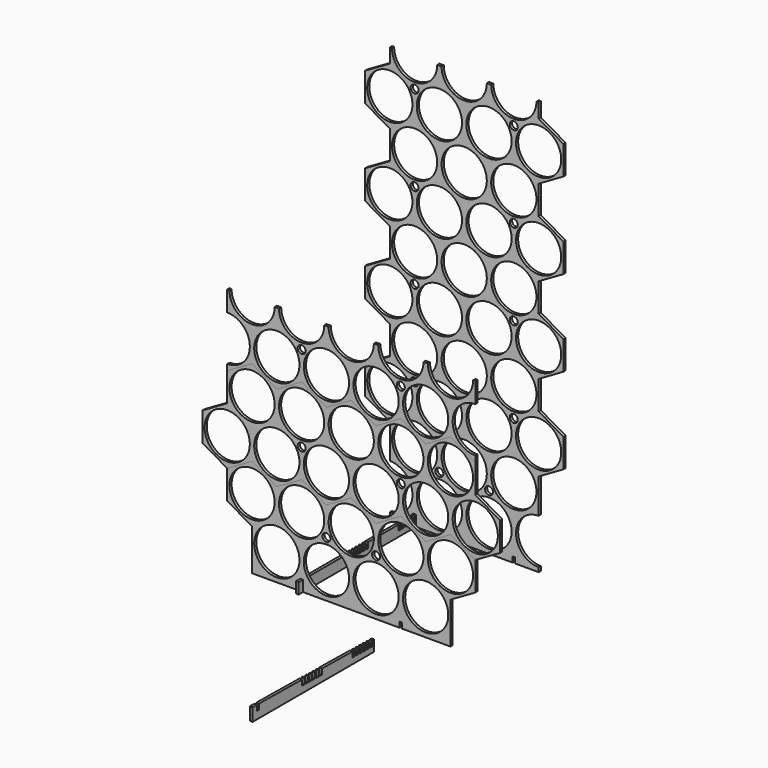
from build123d import *
from build123d import SkipClean  # not in build123d's __all__

# Parameters (mm, degrees)
F0_R           = 41.5
F1_DEPTH       = 5
F2_R           = 41.5
F3_DEPTH       = 5
F4_R           = 41.5
F5_DEPTH       = 5
F10_DEPTH      = 5
F11_R          = 41.5
F12_DEPTH      = 5
F13_R          = 7.25
F14_DEPTH      = 10.001
F14_DEPTH_BACK = 269.001
F16_DEPTH      = 5


with BuildPart() as f1:
    # F0 (on Front) → F1 (new body)
    with BuildSketch(Plane.XZ):
        with BuildLine():
            Line((-88.5, 0), (0, 0))
            Line((0, 0), (0, 86.8083117444))
            ThreePointArc((0, 86.8083117444), (-41.5, 128.3083117444), (0, 169.8083117444))
            Line((0, 169.8083117444), (0, 180.8471862406))
            Line((0, 180.8471862406), (-45.5, 154.5777489925))
            Line((-45.5, 154.5777489925), (-91, 180.8471862406))
            Line((-91, 180.8471862406), (-136.5, 154.5777489925))
            Line((-136.5, 154.5777489925), (-182, 180.8471862406))
            Line((-182, 180.8471862406), (-227.5, 154.5777489925))
            Line((-227.5, 154.5777489925), (-227.5, 102.0388744963))
            Line((-227.5, 102.0388744963), (-182, 75.7694372481))
            Line((-182, 75.7694372481), (-182, 0))
            Line((-182, 0), (-93.5, 0))
            Line((-93.5, 0), (-93.5, 10))
            Line((-93.5, 10), (-88.5, 10))
            Line((-88.5, 10), (-88.5, 0))
        make_face()
        with Locations((-136.5, 49.5)):
            Circle(F0_R, mode=Mode.SUBTRACT)
        with Locations((-45.5, 49.5)):
            Circle(F0_R, mode=Mode.SUBTRACT)
        with Locations((-182, 128.3083117444)):
            Circle(F0_R, mode=Mode.SUBTRACT)
        with Locations((-91, 128.3083117444)):
            Circle(F0_R, mode=Mode.SUBTRACT)
    extrude(amount=F1_DEPTH)

    # F6: F1 across plane


with BuildPart() as f3:
    # F2 (on Front) → F3 (new body)
    with BuildSketch(Plane.XZ):
        with BuildLine():
            Line((-91, 180.8471862406), (-45.5, 154.5777489925))
            Line((-45.5, 154.5777489925), (0, 180.8471862406))
            Line((0, 180.8471862406), (0, 244.4249352332))
            ThreePointArc((0, 244.4249352332), (-41.5, 285.9249352332), (0, 327.4249352332))
            Line((0, 327.4249352332), (0, 338.4638097294))
            Line((0, 338.4638097294), (-45.5, 312.1943724813))
            Line((-45.5, 312.1943724813), (-91, 338.4638097294))
            Line((-91, 338.4638097294), (-136.5, 312.1943724813))
            Line((-136.5, 312.1943724813), (-182, 338.4638097294))
            Line((-182, 338.4638097294), (-227.5, 312.1943724813))
            Line((-227.5, 312.1943724813), (-227.5, 259.655497985))
            Line((-227.5, 259.655497985), (-273, 233.3860607369))
            Line((-273, 233.3860607369), (-273, 180.8471862406))
            Line((-273, 180.8471862406), (-227.5, 154.5777489925))
            Line((-227.5, 154.5777489925), (-182, 180.8471862406))
            Line((-182, 180.8471862406), (-136.5, 154.5777489925))
            Line((-136.5, 154.5777489925), (-91, 180.8471862406))
        make_face()
        with Locations((-227.5, 207.1166234888)):
            Circle(F2_R, mode=Mode.SUBTRACT)
        with Locations((-136.5, 207.1166234888)):
            Circle(F2_R, mode=Mode.SUBTRACT)
        with Locations((-45.5, 207.1166234888)):
            Circle(F2_R, mode=Mode.SUBTRACT)
        with Locations((-182, 285.9249352332)):
            Circle(F2_R, mode=Mode.SUBTRACT)
        with Locations((-91, 285.9249352332)):
            Circle(F2_R, mode=Mode.SUBTRACT)
    extrude(amount=F3_DEPTH)

    # F7: F3 across plane


with BuildPart() as f5:
    # F4 (on Front) → F5 (new body)
    with BuildSketch(Plane.XZ):
        with BuildLine():
            ThreePointArc((-227.5, 406.2332469775), (-186, 364.7332469775), (-227.5, 323.2332469775))
            Line((-227.5, 323.2332469775), (-227.5, 312.1943724813))
            Line((-227.5, 312.1943724813), (-182, 338.4638097294))
            Line((-182, 338.4638097294), (-136.5, 312.1943724813))
            Line((-136.5, 312.1943724813), (-91, 338.4638097294))
            Line((-91, 338.4638097294), (-45.5, 312.1943724813))
            Line((-45.5, 312.1943724813), (0, 338.4638097294))
            Line((0, 338.4638097294), (0, 402.0415587219))
            ThreePointArc((0, 402.0415587219), (-29.3449314192, 414.1966273027), (-41.5, 443.5415587219))
            Line((-41.5, 443.5415587219), (-49.5, 443.5415587219))
            ThreePointArc((-49.5, 443.5415587219), (-91, 402.0415587219), (-132.5, 443.5415587219))
            Line((-132.5, 443.5415587219), (-140.5, 443.5415587219))
            ThreePointArc((-140.5, 443.5415587219), (-182, 402.0415587219), (-223.5, 443.5415587219))
            Line((-223.5, 443.5415587219), (-227.5, 443.5415587219))
            Line((-227.5, 443.5415587219), (-227.5, 406.2332469775))
        make_face()
        with Locations((-136.5, 364.7332469775)):
            Circle(F4_R, mode=Mode.SUBTRACT)
        with Locations((-45.5, 364.7332469775)):
            Circle(F4_R, mode=Mode.SUBTRACT)
    extrude(amount=F5_DEPTH)

    # F8: F5 across plane


with BuildPart() as f1_1:
    add(f1.part, clean=False)
    with SkipClean():  # cleaning this boolean's faces spoils the solid; the shape is the same uncleaned
        add(f1.part.mirror(Plane.YZ), clean=False)


with BuildPart() as f3_1:
    add(f3.part, clean=False)
    with SkipClean():  # cleaning this boolean's faces spoils the solid; the shape is the same uncleaned
        add(f3.part.mirror(Plane.YZ), clean=False)


with BuildPart() as f5_1:
    add(f5.part, clean=False)
    add(f5.part.mirror(Plane.YZ), clean=False)


with BuildPart() as f10:
    # F9 (on face) → F10 (new body)
    with BuildSketch(Plane.YZ.offset(-93.5)):
        Polygon((-15, 20), (-15, 0), (264, 0), (264, 20), (259, 20), (259, 10), (254, 10), (254, 20), (251, 20), (251, 10), (246, 10), (246, 20), (243, 20), (243, 10), (238, 10), (238, 20), (235, 20), (235, 10), (230, 10), (230, 20), (227, 20), (227, 10), (222, 10), (222, 20), (219, 20), (219, 10), (214, 10), (214, 20), (144, 20), (144, 10), (139, 10), (139, 20), (136, 20), (136, 10), (131, 10), (131, 20), (128, 20), (128, 10), (123, 10), (123, 20), (120, 20), (120, 10), (115, 10), (115, 20), (112, 20), (112, 10), (107, 10), (107, 20), (104, 20), (104, 10), (99, 10), (99, 20), (0, 20), (0, 10), (-5, 10), (-5, 20), align=None)
    extrude(amount=F10_DEPTH)


with BuildPart() as f12:
    # F11 (on face) → F12 (new body)
    with BuildSketch(Plane.XZ.offset(-259)):
        with BuildLine():
            Line((-88.5, 0), (88.5, 0))
            Line((88.5, 0), (88.5, 10))
            Line((88.5, 10), (93.5, 10))
            Line((93.5, 10), (93.5, 0))
            Line((93.5, 0), (136.5, 0))
            Line((136.5, 0), (136.5, 8))
            ThreePointArc((136.5, 8), (95, 49.5), (136.5, 91))
            Line((136.5, 91), (136.5, 154.5777489925))
            Line((136.5, 154.5777489925), (182, 180.8471862406))
            Line((182, 180.8471862406), (182, 233.3860607369))
            Line((182, 233.3860607369), (136.5, 259.655497985))
            Line((136.5, 259.655497985), (136.5, 312.1943724813))
            Line((136.5, 312.1943724813), (182, 338.4638097294))
            Line((182, 338.4638097294), (182, 391.0026842257))
            Line((182, 391.0026842257), (136.5, 417.2721214738))
            Line((136.5, 417.2721214738), (136.5, 469.81099597))
            Line((136.5, 469.81099597), (182, 496.0804332182))
            Line((182, 496.0804332182), (182, 548.6193077144))
            Line((182, 548.6193077144), (136.5, 574.8887449626))
            Line((136.5, 574.8887449626), (136.5, 627.4276194588))
            Line((136.5, 627.4276194588), (182, 653.6970567069))
            Line((182, 653.6970567069), (182, 706.2359312032))
            Line((182, 706.2359312032), (136.5, 732.5053684513))
            Line((136.5, 732.5053684513), (136.5, 758.7748056995))
            Line((136.5, 758.7748056995), (132.5, 758.7748056995))
            ThreePointArc((132.5, 758.7748056995), (91, 717.2748056995), (49.5, 758.7748056995))
            Line((49.5, 758.7748056995), (41.5, 758.7748056995))
            ThreePointArc((41.5, 758.7748056995), (0, 717.2748056995), (-41.5, 758.7748056995))
            Line((-41.5, 758.7748056995), (-49.5, 758.7748056995))
            ThreePointArc((-49.5, 758.7748056995), (-91, 717.2748056995), (-132.5, 758.7748056995))
            Line((-132.5, 758.7748056995), (-136.5, 758.7748056995))
            Line((-136.5, 758.7748056995), (-136.5, 732.5053684513))
            Line((-136.5, 732.5053684513), (-182, 706.2359312032))
            Line((-182, 706.2359312032), (-182, 653.6970567069))
            Line((-182, 653.6970567069), (-136.5, 627.4276194588))
            Line((-136.5, 627.4276194588), (-136.5, 574.8887449626))
            Line((-136.5, 574.8887449626), (-182, 548.6193077144))
            Line((-182, 548.6193077144), (-182, 496.0804332182))
            Line((-182, 496.0804332182), (-136.5, 469.81099597))
            Line((-136.5, 469.81099597), (-136.5, 417.2721214738))
            Line((-136.5, 417.2721214738), (-182, 391.0026842257))
            Line((-182, 391.0026842257), (-182, 338.4638097294))
            Line((-182, 338.4638097294), (-136.5, 312.1943724813))
            Line((-136.5, 312.1943724813), (-136.5, 259.655497985))
            Line((-136.5, 259.655497985), (-182, 233.3860607369))
            Line((-182, 233.3860607369), (-182, 180.8471862406))
            Line((-182, 180.8471862406), (-136.5, 154.5777489925))
            Line((-136.5, 154.5777489925), (-136.5, 91))
            ThreePointArc((-136.5, 91), (-95, 49.5), (-136.5, 8))
            Line((-136.5, 8), (-136.5, 0))
            Line((-136.5, 0), (-93.5, 0))
            Line((-93.5, 0), (-93.5, 10))
            Line((-93.5, 10), (-88.5, 10))
            Line((-88.5, 10), (-88.5, 0))
        make_face()
        with Locations((-45.5, 49.5)):
            Circle(F11_R, mode=Mode.SUBTRACT)
        with Locations((-91, 128.3083117444)):
            Circle(F11_R, mode=Mode.SUBTRACT)
        with Locations((-136.5, 207.1166234888)):
            Circle(F11_R, mode=Mode.SUBTRACT)
        with Locations((-136.5, 364.7332469775)):
            Circle(F11_R, mode=Mode.SUBTRACT)
        with Locations((-45.5, 207.1166234888)):
            Circle(F11_R, mode=Mode.SUBTRACT)
        with Locations((-91, 285.9249352332)):
            Circle(F11_R, mode=Mode.SUBTRACT)
        with Locations((-45.5, 364.7332469775)):
            Circle(F11_R, mode=Mode.SUBTRACT)
        with Locations((45.5, 49.5)):
            Circle(F11_R, mode=Mode.SUBTRACT)
        with Locations((0, 128.3083117444)):
            Circle(F11_R, mode=Mode.SUBTRACT)
        with Locations((91, 128.3083117444)):
            Circle(F11_R, mode=Mode.SUBTRACT)
        with Locations((45.5, 207.1166234888)):
            Circle(F11_R, mode=Mode.SUBTRACT)
        with Locations((0, 285.9249352332)):
            Circle(F11_R, mode=Mode.SUBTRACT)
        with Locations((45.5, 364.7332469775)):
            Circle(F11_R, mode=Mode.SUBTRACT)
        with Locations((136.5, 207.1166234888)):
            Circle(F11_R, mode=Mode.SUBTRACT)
        with Locations((91, 285.9249352332)):
            Circle(F11_R, mode=Mode.SUBTRACT)
        with Locations((136.5, 364.7332469775)):
            Circle(F11_R, mode=Mode.SUBTRACT)
        with Locations((-136.5, 522.3498704663)):
            Circle(F11_R, mode=Mode.SUBTRACT)
        with Locations((-91, 443.5415587219)):
            Circle(F11_R, mode=Mode.SUBTRACT)
        with Locations((-45.5, 522.3498704663)):
            Circle(F11_R, mode=Mode.SUBTRACT)
        with Locations((-136.5, 679.9664939551)):
            Circle(F11_R, mode=Mode.SUBTRACT)
        with Locations((-91, 601.1581822107)):
            Circle(F11_R, mode=Mode.SUBTRACT)
        with Locations((-45.5, 679.9664939551)):
            Circle(F11_R, mode=Mode.SUBTRACT)
        with Locations((0, 443.5415587219)):
            Circle(F11_R, mode=Mode.SUBTRACT)
        with Locations((45.5, 522.3498704663)):
            Circle(F11_R, mode=Mode.SUBTRACT)
        with Locations((91, 443.5415587219)):
            Circle(F11_R, mode=Mode.SUBTRACT)
        with Locations((136.5, 522.3498704663)):
            Circle(F11_R, mode=Mode.SUBTRACT)
        with Locations((0, 601.1581822107)):
            Circle(F11_R, mode=Mode.SUBTRACT)
        with Locations((45.5, 679.9664939551)):
            Circle(F11_R, mode=Mode.SUBTRACT)
        with Locations((91, 601.1581822107)):
            Circle(F11_R, mode=Mode.SUBTRACT)
        with Locations((136.5, 679.9664939551)):
            Circle(F11_R, mode=Mode.SUBTRACT)
    extrude(amount=F12_DEPTH)


with BuildPart() as f14_tool:
    # F13 (on face) → F14 (new body, two sides)
    with BuildSketch(Plane.XZ.offset(-254)) as f14_sk:
        with Locations((-45.5, 102.0388744963)):
            Circle(F13_R)
        with Locations((45.5, 102.0388744963)):
            Circle(F13_R)
        with Locations((-91, 233.3860607369)):
            Circle(F13_R)
        with Locations((91, 233.3860607369)):
            Circle(F13_R)
        with Locations((-91, 391.0026842257)):
            Circle(F13_R)
        with Locations((91, 391.0026842257)):
            Circle(F13_R)
        with Locations((-91, 548.6193077144)):
            Circle(F13_R)
        with Locations((91, 548.6193077144)):
            Circle(F13_R)
        with Locations((-91, 706.2359312032)):
            Circle(F13_R)
        with Locations((91, 706.2359312032)):
            Circle(F13_R)
    extrude(amount=-F14_DEPTH)
    extrude(f14_sk.sketch, amount=F14_DEPTH_BACK)


with BuildPart() as f1_2:
    add(f1_1.part, clean=False)

    # F14: cut by f14_tool
    add(f14_tool.part, mode=Mode.SUBTRACT)


with BuildPart() as f3_2:
    add(f3_1.part, clean=False)

    # F14: cut by f14_tool
    add(f14_tool.part, mode=Mode.SUBTRACT)


with BuildPart() as f5_2:
    add(f5_1.part, clean=False)

    # F14: cut by f14_tool
    add(f14_tool.part, mode=Mode.SUBTRACT)


with BuildPart() as f12_1:
    add(f12.part, clean=False)

    # F14: cut by f14_tool
    add(f14_tool.part, mode=Mode.SUBTRACT)


with BuildPart() as f16:
    # F15 (on Right) → F16 (new body)
    with BuildSketch(Plane.YZ):
        Polygon((-227.6199795943, -71.0826882857), (-227.6199795943, -61.0826882857), (-237.6199795943, -60.9455178439), (-237.46979646, -75.0423697711), (41.3767281176, -84.7799049795), (41.3767281176, -64.7725280098), (36.3771984444, -64.7039492403), (36.3771984444, -74.7039492403), (31.3771984444, -74.6353640194), (31.3771984444, -64.6353640194), (28.3774806406, -64.5942167578), (28.3774806406, -74.5942167578), (23.3774806406, -74.5256315369), (23.3774806406, -64.5256315369), (20.3777628367, -64.4844842753), (20.3777628367, -74.4844842753), (15.3777628367, -74.4158990544), (15.3777628367, -64.4158990544), (12.3780450328, -64.3747517927), (12.3780450328, -74.3747517927), (7.3780450328, -74.3061665718), (7.3780450328, -64.3061665718), (4.378327229, -64.2650193102), (4.378327229, -74.2650193102), (-0.621672771, -74.1964340893), (-0.621672771, -64.1964340893), (-3.6213905749, -64.1552868276), (-3.6213905749, -74.1552868276), (-8.6213905749, -74.0867016067), (-8.6213905749, -64.0867016067), (-78.6213905749, -63.1265085141), (-78.6213905749, -73.1265085141), (-83.6213905749, -73.0579232932), (-83.6213905749, -63.0579232932), (-86.6211083788, -63.0167760315), (-86.6211083788, -73.0167760315), (-91.6211083788, -72.9481908106), (-91.6211083788, -62.9481908106), (-94.6208261827, -62.907043549), (-94.6208261827, -72.907043549), (-99.6208261827, -72.8384583281), (-99.6208261827, -62.8384583281), (-102.6205439865, -62.7973110664), (-102.6205439865, -72.7973110664), (-107.6205439865, -72.7287258455), (-107.6205439865, -62.7287258455), (-110.6202617904, -62.6875785839), (-110.6202617904, -72.6875785839), (-115.6202617904, -72.618993363), (-115.6202617904, -62.618993363), (-118.6199795943, -62.5778461014), (-118.6199795943, -72.5778461014), (-123.6199795943, -72.5092608805), (-123.6199795943, -62.5092608805), (-222.6199795943, -61.1512735066), (-222.6199795943, -71.1512735066), align=None)
        Polygon((41.3767281176, -84.7799049795), (-237.46979646, -75.0423697711), (-237.3660560245, -84.7799049795), align=None)
    extrude(amount=F16_DEPTH)


solid = Compound([f10.part, f1_2.part, f3_2.part, f5_2.part, f12_1.part, f16.part])
